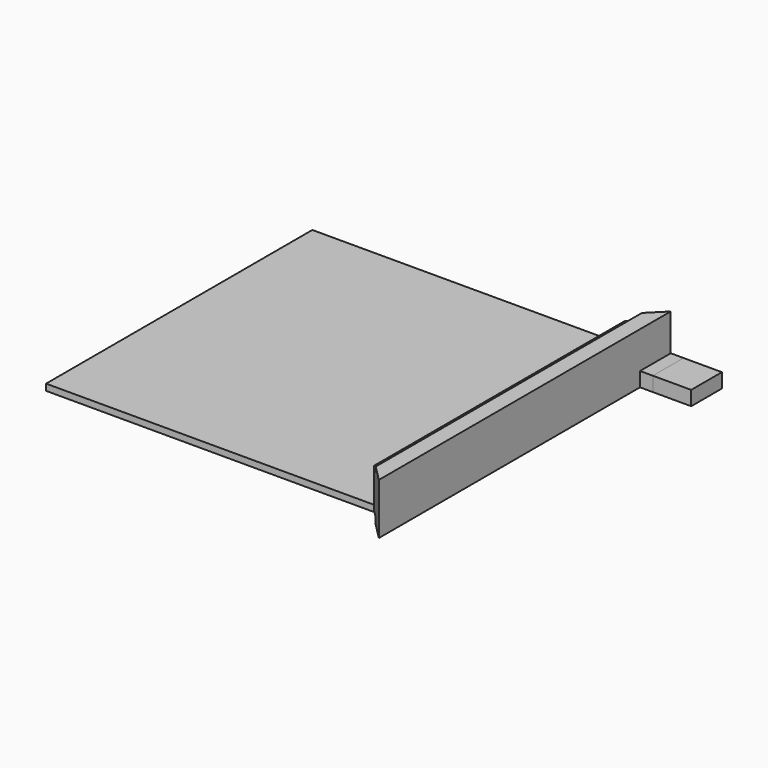
from build123d import *

# Parameters (mm, degrees)
F0_W      = 330.2
F0_H      = 330.2
F3_DEPTH  = 6.35
F2_W      = 38.1
F2_H      = 38.1
F4_DEPTH  = 14.2875
F1_W      = 25.4
F1_H      = 50.8
F5_DEPTH  = 361.95
F8_SIZE   = 25.39999
F6_W      = 9.525
F6_H      = 6.35
F9_DEPTH  = 361.951
F7_W      = 3.175
F7_H      = 14.2875
F10_DEPTH = 307.975
F11_W     = 38.1
F11_H     = 38.1
F12_DEPTH = 14.2875


# Not quite as in the source:
# - a fillet or chamfer is up to 0.001 mm smaller than in the source, because OpenCascade refuses the exact size


with BuildPart() as f3:
    # F0 (on Top) → F3 (new body)
    with BuildSketch(Plane.XY):
        with Locations((-165.1, -165.1)):
            Rectangle(F0_W, F0_H)
    extrude(amount=F3_DEPTH)


with BuildPart() as f4:
    # F2 (on Top) → F4 (new body)
    with BuildSketch(Plane.XY):
        with Locations((19.05, -19.05)):
            Rectangle(F2_W, F2_H)
    extrude(amount=F4_DEPTH)


with BuildPart() as f5:
    # F1 (on Front) → F5 (new body)
    with BuildSketch(Plane.XZ):
        with Locations((12.7, 25.4)):
            Rectangle(F1_W, F1_H)
    extrude(amount=F5_DEPTH)

    # F8 (size 25.4 in the source; OpenCascade refuses exactly that, so slightly less here)
    f8_edges = [f5.edges().sort_by_distance(p)[0] for p in [
        (0, -361.95, 25.4),
        (0, 0, 25.4),
    ]]
    chamfer(f8_edges, length=F8_SIZE)

    # F6 (on face) → F9 (cut, through all)
    with BuildSketch(Plane.XZ.offset(361.95)):
        with Locations((4.7625, 47.625)):
            Rectangle(F6_W, F6_H)
        with Locations((4.7625, 3.175)):
            Rectangle(F6_W, F6_H)
    extrude(amount=-F9_DEPTH, mode=Mode.SUBTRACT)


with BuildPart() as f10:
    # F7 (on Front) → F10 (new body)
    with BuildSketch(Plane.XZ):
        with Locations((-1.5875, 17.2649201432)):
            Rectangle(F7_W, F7_H)
    extrude(amount=F10_DEPTH)


with BuildPart() as f12:
    # F11 (on Top) → F12 (new body)
    with BuildSketch(Plane.XY):
        with Locations((57.15, -19.05)):
            Rectangle(F11_W, F11_H)
    extrude(amount=F12_DEPTH)


solid = Compound([f3.part, f4.part, f5.part, f10.part, f12.part])
